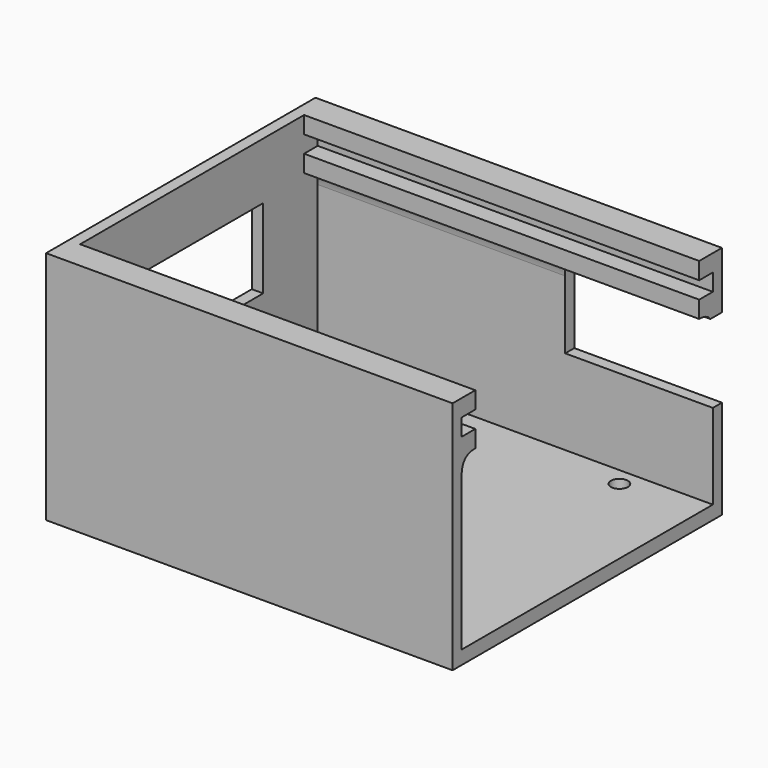
from build123d import *

# Parameters (mm, degrees)
F1_W        = 68.6
F1_H        = 53.3
F1_R        = 1.5
F2_DEPTH    = 2.4
F4_DEPTH    = 39
F6_DEPTH    = 69.6
F7_T1_DEPTH = 69.6
F8_W        = 29.3
F8_H        = 14
F9_DEPTH    = 25.4
F10_W       = 26
F10_H       = 14
F11_DEPTH   = 25.4


# Not quite as in the source:
# - a fillet or chamfer that OpenCascade refuses, or shapes differently, is made with other operations: its cross-section is extruded or revolved along the edge and cut away or added


with BuildPart() as f2:
    # F1 (on Top) → F2 (new body)
    with BuildSketch(Plane.XY):
        Polygon((-68.6, 0), (-68.6, 53.3), (0, 53.3), (0, 56.3), (-71.6, 56.3), (-71.6, -3), (0, -3), (0, 0), align=None)
        with Locations((-34.3, 26.65)):
            Rectangle(F1_W, F1_H)
        with Locations((-66.4, 7.9)):
            Circle(F1_R, mode=Mode.SUBTRACT)
        with Locations((-15.2, 2.2)):
            Circle(F1_R, mode=Mode.SUBTRACT)
        with Locations((-66.3, 35.8)):
            Circle(F1_R, mode=Mode.SUBTRACT)
        with Locations((-13.9, 51.1)):
            Circle(F1_R, mode=Mode.SUBTRACT)
    extrude(amount=F2_DEPTH)

    # F3 (on face) → F4 (join)
    with BuildSketch(Plane.XY.offset(2.4)):
        Polygon((0, 54.3), (0, 56.3), (-71.6, 56.3), (-71.6, -3), (0, -3), (0, -1), (-69.6, -1), (-69.6, 54.3), align=None)
    extrude(amount=F4_DEPTH)

    # F5 (on face) → F6 (join, through all)
    with BuildSketch(Plane.YZ.offset(-69.6)):
        Polygon((2, 41.4), (-1, 41.4), (-2.3718131706, 41.4), (-2.3718131706, 32.4), (-1, 32.4), (2, 32.4), (2, 35.4), (-1, 35.4), (-1, 38.4), (2, 38.4), align=None)
        Polygon((55.6718131706, 32.4), (55.6718131706, 41.4), (54.3, 41.4), (51.3, 41.4), (51.3, 38.4), (54.3, 38.4), (54.3, 35.4), (51.3, 35.4), (51.3, 32.4), (54.3, 32.4), align=None)
    extrude(amount=F6_DEPTH)

    # F7: fillet of radius 3 on 2 edges, made by hand

    # F7_s2 → F7_t1 (join)
    with BuildSketch(Plane.YZ.offset(-69.6)):
        with BuildLine():
            add(Edge.make_bspline(
                [(2, 32.4), (-1, 32.4), (-1, 29.4)],
                knots=[0, 0, 0, 1, 1, 1], degree=2, weights=[1, 1, 1]))
            Line((-1, 29.4), (-1, 32.4))
            Line((-1, 32.4), (2, 32.4))
        make_face()
        with BuildLine():
            add(Edge.make_bspline(
                [(54.3, 29.4), (54.3, 32.4), (51.3, 32.4)],
                knots=[0, 0, 0, 1, 1, 1], degree=2, weights=[1, 1, 1]))
            Line((51.3, 32.4), (54.3, 32.4))
            Line((54.3, 32.4), (54.3, 29.4))
        make_face()
    extrude(amount=F7_T1_DEPTH)

    # F8 (on face) → F9 (cut)
    with BuildSketch(Plane.YZ.offset(-69.6)):
        with Locations((27.65, 24.4)):
            Rectangle(F8_W, F8_H)
    extrude(amount=-F9_DEPTH, mode=Mode.SUBTRACT)

    # F10 (on face) → F11 (cut)
    with BuildSketch(Plane(origin=(0, 56.3, 0), x_dir=(-1, 0, 0), z_dir=(0, 1, 0))):
        with Locations((13, 24.4)):
            Rectangle(F10_W, F10_H)
    extrude(amount=-F11_DEPTH, mode=Mode.SUBTRACT)


solid = f2.part
